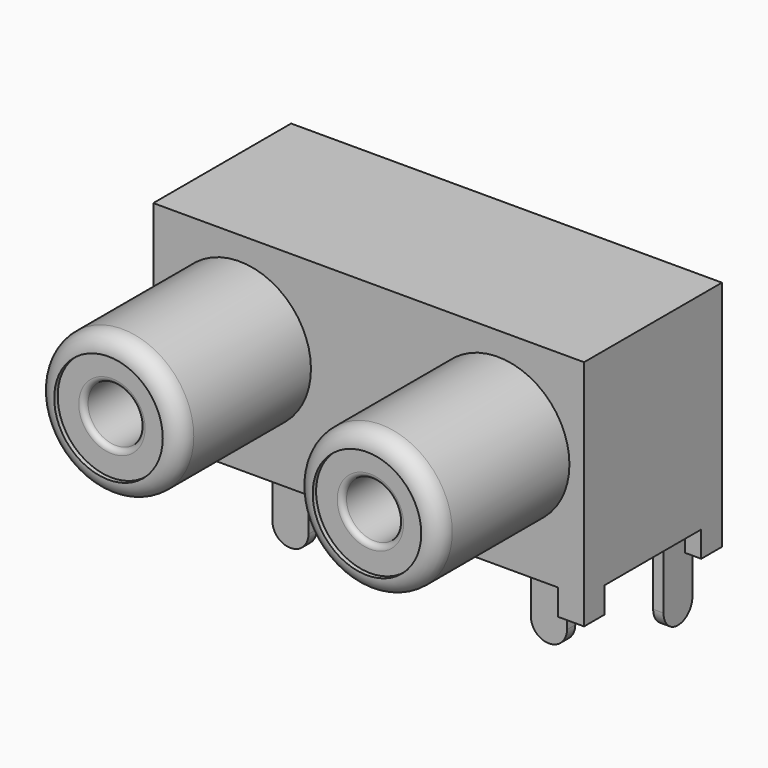
from build123d import *

# Parameters (mm, degrees)
F0_R           = 4.15
F0_R_2         = 3.15
F1_DEPTH       = 9.5
F0_R_3         = 1.625
F2_DEPTH       = 9.25
F3_R           = 0.99999
F3_2_R         = 0.99999
F4_DEPTH       = 10
F6_W           = 7
F6_H           = 1.5
F7_DEPTH       = 25
F10_DEPTH      = 0.3
F10_DEPTH_BACK = 0.3
F19_DEPTH      = 0.3
F19_DEPTH_BACK = 0.3
F20_R          = 0.3
F20_2_R        = 0.3


# Not quite as in the source:
# - a fillet or chamfer is up to 0.001 mm smaller than in the source, because OpenCascade refuses the exact size


with BuildPart() as f1:
    # F0 (on Front) → F1 (new body)
    with BuildSketch(Plane.XZ):
        with Locations((-7.5, 0)):
            Circle(F0_R)
        with Locations((-7.5, 0)):
            Circle(F0_R_2, mode=Mode.SUBTRACT)
    extrude(amount=F1_DEPTH)

    # F3 (radius 1 in the source; OpenCascade refuses exactly that, so slightly less here)
    f3_edges = [f1.edges().sort_by_distance(p)[0] for p in [
        (-11.65, -9.5, 0),
    ]]
    fillet(f3_edges, radius=F3_R)


with BuildPart() as f1b:
    # F0 (on Front) → F1, piece 2 (new body)
    with BuildSketch(Plane.XZ):
        with Locations((7.5, 0)):
            Circle(F0_R)
        with Locations((7.5, 0)):
            Circle(F0_R_2, mode=Mode.SUBTRACT)
    extrude(amount=F1_DEPTH)

    # F3#2 (radius 1 in the source; OpenCascade refuses exactly that, so slightly less here)
    f3_2_edges = [f1b.edges().sort_by_distance(p)[0] for p in [
        (3.35, -9.5, 0),
    ]]
    fillet(f3_2_edges, radius=F3_2_R)


with BuildPart() as f2:
    # F0 (on Front) → F2 (new body)
    with BuildSketch(Plane.XZ):
        with Locations((-7.5, 0)):
            Circle(F0_R_2)
        with Locations((-7.5, 0)):
            Circle(F0_R_3, mode=Mode.SUBTRACT)
    extrude(amount=F2_DEPTH)

    # F20
    f20_edges = [f2.edges().sort_by_distance(p)[0] for p in [
        (-9.125, -9.25, 0),
    ]]
    fillet(f20_edges, radius=F20_R)


with BuildPart() as f2b:
    # F0 (on Front) → F2, piece 2 (new body)
    with BuildSketch(Plane.XZ):
        with Locations((7.5, 0)):
            Circle(F0_R_2)
        with Locations((7.5, 0)):
            Circle(F0_R_3, mode=Mode.SUBTRACT)
    extrude(amount=F2_DEPTH)

    # F20#2
    f20_2_edges = [f2b.edges().sort_by_distance(p)[0] for p in [
        (5.875, -9.25, 0),
    ]]
    fillet(f20_2_edges, radius=F20_2_R)


with BuildPart() as f4:
    # F0 (on Front) → F4 (new body)
    with BuildSketch(Plane.XZ):
        Polygon((12.5, 5.5), (-12.5, 5.5), (-12.5, -8), (-11, -8), (-11, -6.5), (11, -6.5), (11, -8), (12.5, -8), align=None)
        with Locations((-7.5, 0)):
            Circle(F0_R, mode=Mode.SUBTRACT)
        with Locations((7.5, 0)):
            Circle(F0_R, mode=Mode.SUBTRACT)
        with Locations((7.5, 0)):
            Circle(F0_R)
        with Locations((7.5, 0)):
            Circle(F0_R_2, mode=Mode.SUBTRACT)
        with Locations((-7.5, 0)):
            Circle(F0_R)
        with Locations((-7.5, 0)):
            Circle(F0_R_2, mode=Mode.SUBTRACT)
        with Locations((7.5, 0)):
            Circle(F0_R_2)
        with Locations((7.5, 0)):
            Circle(F0_R_3, mode=Mode.SUBTRACT)
        with Locations((-7.5, 0)):
            Circle(F0_R_2)
        with Locations((-7.5, 0)):
            Circle(F0_R_3, mode=Mode.SUBTRACT)
        with Locations((7.5, 0)):
            Circle(F0_R_3)
        with Locations((-7.5, 0)):
            Circle(F0_R_3)
    extrude(amount=-F4_DEPTH)

    # F6 (on offset) → F7 (cut)
    with BuildSketch(Plane.YZ.offset(12.5)):
        with Locations((5, -7.25)):
            Rectangle(F6_W, F6_H)
    extrude(amount=-F7_DEPTH, mode=Mode.SUBTRACT)


with BuildPart() as f10:
    # F9 (on offset) → F10 (new body, two sides)
    with BuildSketch(Plane.XZ.offset(-4)) as f10_sk:
        with BuildLine():
            Line((-6.45, -10.95), (-6.45, -4.5750031686))
            Line((-6.45, -4.5750031686), (-8.55, -4.5750031686))
            Line((-8.55, -4.5750031686), (-8.55, -10.95))
            ThreePointArc((-8.55, -10.95), (-7.5, -12), (-6.45, -10.95))
        make_face()
    extrude(amount=F10_DEPTH)
    extrude(f10_sk.sketch, amount=-F10_DEPTH_BACK)


with BuildPart() as f10b:
    # F9 (on offset) → F10, piece 2 (new body, two sides)
    with BuildSketch(Plane.XZ.offset(-4)) as f10_2_sk:
        with BuildLine():
            ThreePointArc((6.45, -10.95), (7.5, -12), (8.55, -10.95))
            Line((8.55, -10.95), (8.55, -4.5750031686))
            Line((8.55, -4.5750031686), (6.45, -4.5750031686))
            Line((6.45, -4.5750031686), (6.45, -10.95))
        make_face()
    extrude(amount=F10_DEPTH)
    extrude(f10_2_sk.sketch, amount=-F10_DEPTH_BACK)


with BuildPart() as f19:
    # F18 (on offset) → F19 (new body, two sides)
    with BuildSketch(Plane.YZ.offset(-11.25)) as f19_sk:
        with BuildLine():
            Line((9.05, -5.7792608787), (6.95, -5.7792608787))
            Line((6.95, -5.7792608787), (6.95, -10.45))
            ThreePointArc((6.95, -10.45), (8, -11.5), (9.05, -10.45))
            Line((9.05, -10.45), (9.05, -5.7792608787))
        make_face()
    extrude(amount=F19_DEPTH)
    extrude(f19_sk.sketch, amount=-F19_DEPTH_BACK)


with BuildPart() as f19b:
    # F17 (on offset) → F19, piece 2 (new body, two sides)
    with BuildSketch(Plane.YZ.offset(-3.75)) as f19_2_sk:
        with BuildLine():
            Line((9.05, -5.7792608787), (6.95, -5.7792608787))
            Line((6.95, -5.7792608787), (6.95, -10.45))
            ThreePointArc((6.95, -10.45), (8, -11.5), (9.05, -10.45))
            Line((9.05, -10.45), (9.05, -5.7792608787))
        make_face()
    extrude(amount=F19_DEPTH)
    extrude(f19_2_sk.sketch, amount=-F19_DEPTH_BACK)


with BuildPart() as f19c:
    # F16 (on offset) → F19, piece 3 (new body, two sides)
    with BuildSketch(Plane.YZ.offset(3.75)) as f19_3_sk:
        with BuildLine():
            Line((9.05, -5.7792608787), (6.95, -5.7792608787))
            Line((6.95, -5.7792608787), (6.95, -10.45))
            ThreePointArc((6.95, -10.45), (8, -11.5), (9.05, -10.45))
            Line((9.05, -10.45), (9.05, -5.7792608787))
        make_face()
    extrude(amount=F19_DEPTH)
    extrude(f19_3_sk.sketch, amount=-F19_DEPTH_BACK)


with BuildPart() as f19d:
    # F15 (on offset) → F19, piece 4 (new body, two sides)
    with BuildSketch(Plane.YZ.offset(11.25)) as f19_4_sk:
        with BuildLine():
            Line((9.05, -5.7792608787), (6.95, -5.7792608787))
            Line((6.95, -5.7792608787), (6.95, -10.45))
            ThreePointArc((6.95, -10.45), (8, -11.5), (9.05, -10.45))
            Line((9.05, -10.45), (9.05, -5.7792608787))
        make_face()
    extrude(amount=F19_DEPTH)
    extrude(f19_4_sk.sketch, amount=-F19_DEPTH_BACK)


solid = Compound([f1.part, f1b.part, f2.part, f2b.part, f4.part, f10.part, f10b.part, f19.part, f19b.part, f19c.part, f19d.part])
